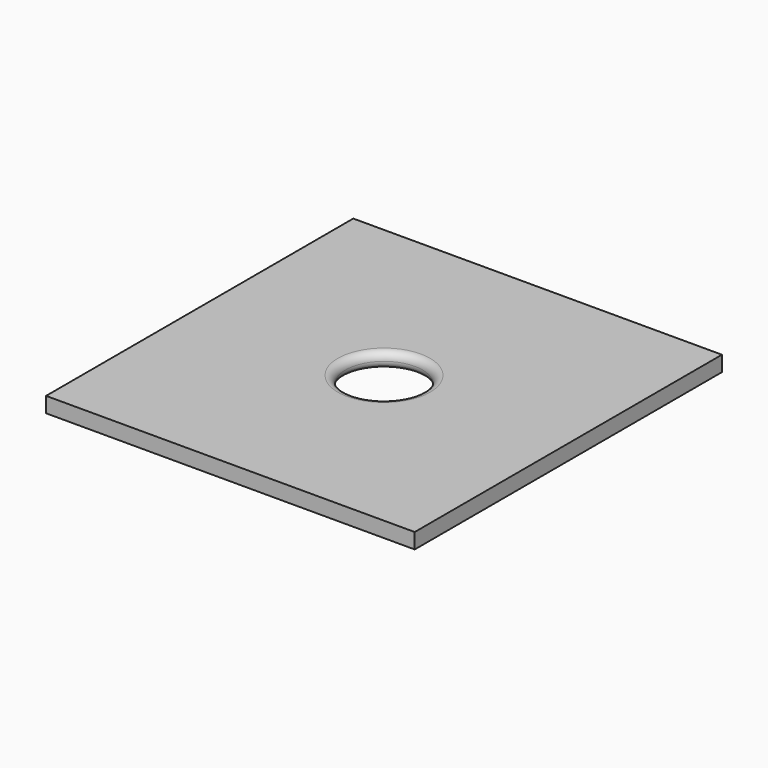
from build123d import *

# Parameters (mm, degrees)
F0_W     = 60.96
F0_H     = 63.5
F0_R     = 6.35
F1_DEPTH = 2.54
F2_R     = 1.26999


# Not quite as in the source:
# - a fillet or chamfer is up to 0.001 mm smaller than in the source, because OpenCascade refuses the exact size


with BuildPart() as f1:
    # F0 (on Top) → F1 (new body)
    with BuildSketch(Plane.XY):
        Rectangle(F0_W, F0_H)
        Circle(F0_R, mode=Mode.SUBTRACT)
    extrude(amount=F1_DEPTH)

    # F2 (radius 1.27 in the source; OpenCascade refuses exactly that, so slightly less here)
    f2_edges = [f1.edges().sort_by_distance(p)[0] for p in [
        (-6.35, 0, 2.54),
        (-6.35, 0, 0),
    ]]
    fillet(f2_edges, radius=F2_R)


solid = f1.part
